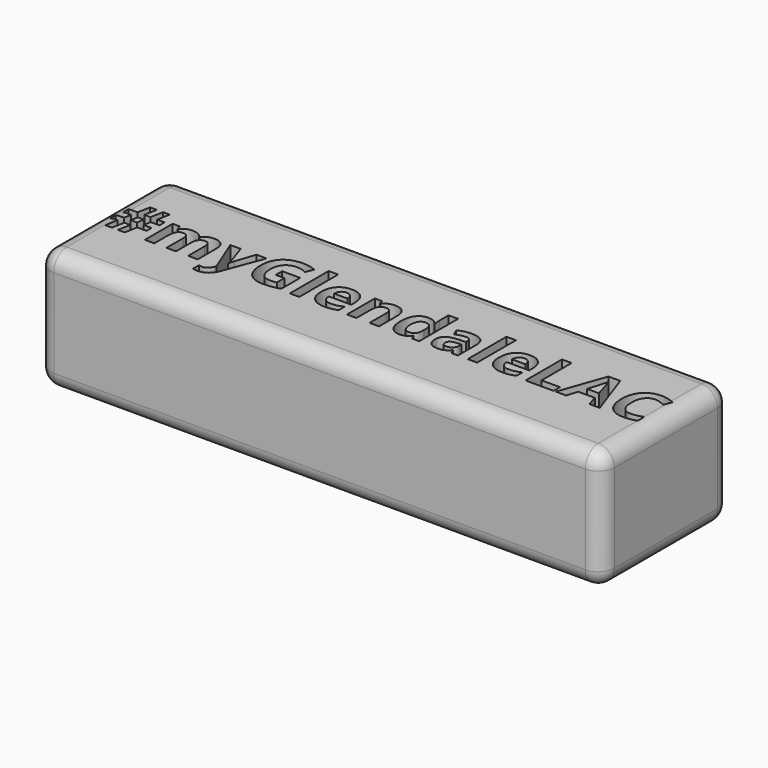
from build123d import *

# Parameters (mm, degrees)
F0_W         = 177.8
F0_H         = 50.8
F1_DEPTH     = 38.1
F2_TEXT_SIZE = 20.1029624608
F3_DEPTH     = 38.1
F4_T1_DEPTH  = 167.64
F4_T3_DEPTH  = 40.64
F4_T5_DEPTH  = 27.94
F4_S9_W      = 5.1816
F4_S9_H      = 5.1816
F4_T10_DEPTH = 5.1816
F4_S15_W     = 5.1816
F4_S15_H     = 5.1816
F4_T16_DEPTH = 5.1816
F4_S21_W     = 5.1816
F4_S21_H     = 5.1816
F4_T22_DEPTH = 5.1816
F4_S27_W     = 5.1816
F4_S27_H     = 5.1816
F4_T28_DEPTH = 5.1816
F4_S33_W     = 5.1816
F4_S33_H     = 5.1816
F4_T34_DEPTH = 5.1816
F4_S39_W     = 5.1816
F4_S39_H     = 5.1816
F4_T40_DEPTH = 5.1816
F4_S45_W     = 5.1816
F4_S45_H     = 5.1816
F4_T46_DEPTH = 5.1816
F4_S51_W     = 5.1816
F4_S51_H     = 5.1816
F4_T52_DEPTH = 5.1816


# Not quite as in the source:
# - a fillet or chamfer that OpenCascade refuses, or shapes differently, is made with other operations: its cross-section is extruded or revolved along the edge and cut away or added
# - Text() gives the source's letters only with a copy of the font that has no kerning and outlines rounded to 1/6400 em; it was checked with that copy


with BuildPart() as f1:
    # F0 (on Top) → F1 (new body)
    with BuildSketch(Plane.XY):
        Rectangle(F0_W, F0_H)
    extrude(amount=F1_DEPTH)

    # F2 (on face) → F3 (cut, through all)
    with BuildSketch(Plane.XY.offset(38.1)):
        with Locations((-85.725, -5.3196763222)):
            Text('#myGlendaleLAC', F2_TEXT_SIZE, font='Open Sans', font_style=FontStyle.BOLD, text_align=(TextAlign.LEFT, TextAlign.BOTTOM))
    extrude(amount=-F3_DEPTH, mode=Mode.SUBTRACT)

    # F4: fillet of radius 5.08 on 12 edges, made by hand

    # F4_s2 → F4_t1 (cut)
    with BuildSketch(Plane.YZ.offset(-83.82)):
        with BuildLine():
            ThreePointArc((25.4, 33.02), (23.9121024484, 36.6121024484), (20.32, 38.1))
            Line((20.32, 38.1), (20.32, 38.2016))
            Line((20.32, 38.2016), (25.5016, 38.2016))
            Line((25.5016, 38.2016), (25.5016, 33.02))
            Line((25.5016, 33.02), (25.4, 33.02))
        make_face()
        with BuildLine():
            ThreePointArc((-25.4, 5.08), (-23.9121024484, 1.4878975516), (-20.32, 0))
            Line((-20.32, 0), (-20.32, -0.1016))
            Line((-20.32, -0.1016), (-25.5016, -0.1016))
            Line((-25.5016, -0.1016), (-25.5016, 5.08))
            Line((-25.5016, 5.08), (-25.4, 5.08))
        make_face()
        with BuildLine():
            ThreePointArc((-25.4, 33.02), (-23.9121024484, 36.6121024484), (-20.32, 38.1))
            Line((-20.32, 38.1), (-20.32, 38.2016))
            Line((-20.32, 38.2016), (-25.5016, 38.2016))
            Line((-25.5016, 38.2016), (-25.5016, 33.02))
            Line((-25.5016, 33.02), (-25.4, 33.02))
        make_face()
        with BuildLine():
            ThreePointArc((25.4, 5.08), (23.9121024484, 1.4878975516), (20.32, 0))
            Line((20.32, 0), (20.32, -0.1016))
            Line((20.32, -0.1016), (25.5016, -0.1016))
            Line((25.5016, -0.1016), (25.5016, 5.08))
            Line((25.5016, 5.08), (25.4, 5.08))
        make_face()
    extrude(amount=F4_T1_DEPTH, mode=Mode.SUBTRACT)

    # F4_s4 → F4_t3 (cut)
    with BuildSketch(Plane.XZ.offset(-20.32)):
        with BuildLine():
            ThreePointArc((-83.82, 38.1), (-87.4121024484, 36.6121024484), (-88.9, 33.02))
            Line((-88.9, 33.02), (-89.0016, 33.02))
            Line((-89.0016, 33.02), (-89.0016, 38.2016))
            Line((-89.0016, 38.2016), (-83.82, 38.2016))
            Line((-83.82, 38.2016), (-83.82, 38.1))
        make_face()
        with BuildLine():
            ThreePointArc((-83.82, 0), (-87.4121024484, 1.4878975516), (-88.9, 5.08))
            Line((-88.9, 5.08), (-89.0016, 5.08))
            Line((-89.0016, 5.08), (-89.0016, -0.1016))
            Line((-89.0016, -0.1016), (-83.82, -0.1016))
            Line((-83.82, -0.1016), (-83.82, 0))
        make_face()
        with BuildLine():
            ThreePointArc((88.9, 5.08), (87.4121024484, 1.4878975516), (83.82, 0))
            Line((83.82, 0), (83.82, -0.1016))
            Line((83.82, -0.1016), (89.0016, -0.1016))
            Line((89.0016, -0.1016), (89.0016, 5.08))
            Line((89.0016, 5.08), (88.9, 5.08))
        make_face()
        with BuildLine():
            ThreePointArc((88.9, 33.02), (87.4121024484, 36.6121024484), (83.82, 38.1))
            Line((83.82, 38.1), (83.82, 38.2016))
            Line((83.82, 38.2016), (89.0016, 38.2016))
            Line((89.0016, 38.2016), (89.0016, 33.02))
            Line((89.0016, 33.02), (88.9, 33.02))
        make_face()
    extrude(amount=F4_T3_DEPTH, mode=Mode.SUBTRACT)

    # F4_s6 → F4_t5 (cut)
    with BuildSketch(Plane.XY.offset(5.08)):
        with BuildLine():
            ThreePointArc((-83.82, 25.4), (-87.4121024484, 23.9121024484), (-88.9, 20.32))
            Line((-88.9, 20.32), (-89.0016, 20.32))
            Line((-89.0016, 20.32), (-89.0016, 25.5016))
            Line((-89.0016, 25.5016), (-83.82, 25.5016))
            Line((-83.82, 25.5016), (-83.82, 25.4))
        make_face()
        with BuildLine():
            ThreePointArc((-83.82, -25.4), (-87.4121024484, -23.9121024484), (-88.9, -20.32))
            Line((-88.9, -20.32), (-89.0016, -20.32))
            Line((-89.0016, -20.32), (-89.0016, -25.5016))
            Line((-89.0016, -25.5016), (-83.82, -25.5016))
            Line((-83.82, -25.5016), (-83.82, -25.4))
        make_face()
        with BuildLine():
            ThreePointArc((88.9, -20.32), (87.4121024484, -23.9121024484), (83.82, -25.4))
            Line((83.82, -25.4), (83.82, -25.5016))
            Line((83.82, -25.5016), (89.0016, -25.5016))
            Line((89.0016, -25.5016), (89.0016, -20.32))
            Line((89.0016, -20.32), (88.9, -20.32))
        make_face()
        with BuildLine():
            ThreePointArc((88.9, 20.32), (87.4121024484, 23.9121024484), (83.82, 25.4))
            Line((83.82, 25.4), (83.82, 25.5016))
            Line((83.82, 25.5016), (89.0016, 25.5016))
            Line((89.0016, 25.5016), (89.0016, 20.32))
            Line((89.0016, 20.32), (88.9, 20.32))
        make_face()
    extrude(amount=F4_T5_DEPTH, mode=Mode.SUBTRACT)


with BuildPart() as f4_tool8:
    # F4_s9 → F4_t10 (new body)
    with BuildSketch(Plane.YZ.offset(83.82)):
        with Locations((22.9108, 35.6108)):
            Rectangle(F4_S9_W, F4_S9_H)
    extrude(amount=F4_T10_DEPTH)

    # F4_s11 → F4_t12 (revolve, cut)
    with BuildSketch(Plane(origin=(83.82, 20.32, 33.02), x_dir=(0, -0.7071067812, -0.7071067812), z_dir=(0, -0.7071067812, 0.7071067812))):
        with BuildLine():
            ThreePointArc((0, -5.08), (5.08, 0), (0, 5.08))
            Line((0, 5.08), (0, -5.08))
        make_face()
    revolve(axis=Axis((83.82, 20.32, 33.02), (1, 0, 0)), mode=Mode.SUBTRACT)


with BuildPart() as f1_1:
    add(f1.part)

    # F4_t7: cut F4_tool8
    add(f4_tool8.part, mode=Mode.SUBTRACT)


with BuildPart() as f4_tool14:
    # F4_s15 → F4_t16 (new body)
    with BuildSketch(Plane.XZ.offset(-20.32)):
        with Locations((-86.4108, 35.6108)):
            Rectangle(F4_S15_W, F4_S15_H)
    extrude(amount=-F4_T16_DEPTH)

    # F4_s17 → F4_t18 (revolve, cut)
    with BuildSketch(Plane(origin=(-83.82, 20.32, 33.02), x_dir=(0.7071067812, 0, -0.7071067812), z_dir=(0.7071067812, 0, 0.7071067812))):
        with BuildLine():
            ThreePointArc((0, -5.08), (5.08, 0), (0, 5.08))
            Line((0, 5.08), (0, -5.08))
        make_face()
    revolve(axis=Axis((-83.82, 20.32, 33.02), (0, 1, 0)), mode=Mode.SUBTRACT)


with BuildPart() as f1_2:
    add(f1_1.part)

    # F4_t13: cut F4_tool14
    add(f4_tool14.part, mode=Mode.SUBTRACT)


with BuildPart() as f4_tool20:
    # F4_s21 → F4_t22 (new body)
    with BuildSketch(Plane.XZ.offset(20.32)):
        with Locations((-86.4108, 35.6108)):
            Rectangle(F4_S21_W, F4_S21_H)
    extrude(amount=F4_T22_DEPTH)

    # F4_s23 → F4_t24 (revolve, cut)
    with BuildSketch(Plane(origin=(-83.82, -20.32, 33.02), x_dir=(0.7071067812, 0, -0.7071067812), z_dir=(-0.7071067812, 0, -0.7071067812))):
        with BuildLine():
            ThreePointArc((0, -5.08), (5.08, 0), (0, 5.08))
            Line((0, 5.08), (0, -5.08))
        make_face()
    revolve(axis=Axis((-83.82, -20.32, 33.02), (0, -1, 0)), mode=Mode.SUBTRACT)


with BuildPart() as f1_3:
    add(f1_2.part)

    # F4_t19: cut F4_tool20
    add(f4_tool20.part, mode=Mode.SUBTRACT)


with BuildPart() as f4_tool26:
    # F4_s27 → F4_t28 (new body)
    with BuildSketch(Plane.XZ.offset(-20.32)):
        with Locations((-86.4108, 2.4892)):
            Rectangle(F4_S27_W, F4_S27_H)
    extrude(amount=-F4_T28_DEPTH)

    # F4_s29 → F4_t30 (revolve, cut)
    with BuildSketch(Plane(origin=(-83.82, 20.32, 5.08), x_dir=(0.7071067812, 0, 0.7071067812), z_dir=(-0.7071067812, 0, 0.7071067812))):
        with BuildLine():
            ThreePointArc((0, -5.08), (5.08, 0), (0, 5.08))
            Line((0, 5.08), (0, -5.08))
        make_face()
    revolve(axis=Axis((-83.82, 20.32, 5.08), (0, 1, 0)), mode=Mode.SUBTRACT)


with BuildPart() as f1_4:
    add(f1_3.part)

    # F4_t25: cut F4_tool26
    add(f4_tool26.part, mode=Mode.SUBTRACT)


with BuildPart() as f4_tool32:
    # F4_s33 → F4_t34 (new body)
    with BuildSketch(Plane.XZ.offset(20.32)):
        with Locations((-86.4108, 2.4892)):
            Rectangle(F4_S33_W, F4_S33_H)
    extrude(amount=F4_T34_DEPTH)

    # F4_s35 → F4_t36 (revolve, cut)
    with BuildSketch(Plane(origin=(-83.82, -20.32, 5.08), x_dir=(0.7071067812, 0, 0.7071067812), z_dir=(0.7071067812, 0, -0.7071067812))):
        with BuildLine():
            ThreePointArc((0, -5.08), (5.08, 0), (0, 5.08))
            Line((0, 5.08), (0, -5.08))
        make_face()
    revolve(axis=Axis((-83.82, -20.32, 5.08), (0, -1, 0)), mode=Mode.SUBTRACT)


with BuildPart() as f1_5:
    add(f1_4.part)

    # F4_t31: cut F4_tool32
    add(f4_tool32.part, mode=Mode.SUBTRACT)


with BuildPart() as f4_tool38:
    # F4_s39 → F4_t40 (new body)
    with BuildSketch(Plane.YZ.offset(83.82)):
        with Locations((-22.9108, 2.4892)):
            Rectangle(F4_S39_W, F4_S39_H)
    extrude(amount=F4_T40_DEPTH)

    # F4_s41 → F4_t42 (revolve, cut)
    with BuildSketch(Plane(origin=(83.82, -20.32, 5.08), x_dir=(0, 0.7071067812, 0.7071067812), z_dir=(0, 0.7071067812, -0.7071067812))):
        with BuildLine():
            ThreePointArc((0, -5.08), (5.08, 0), (0, 5.08))
            Line((0, 5.08), (0, -5.08))
        make_face()
    revolve(axis=Axis((83.82, -20.32, 5.08), (1, 0, 0)), mode=Mode.SUBTRACT)


with BuildPart() as f1_6:
    add(f1_5.part)

    # F4_t37: cut F4_tool38
    add(f4_tool38.part, mode=Mode.SUBTRACT)


with BuildPart() as f4_tool44:
    # F4_s45 → F4_t46 (new body)
    with BuildSketch(Plane.YZ.offset(83.82)):
        with Locations((-22.9108, 35.6108)):
            Rectangle(F4_S45_W, F4_S45_H)
    extrude(amount=F4_T46_DEPTH)

    # F4_s47 → F4_t48 (revolve, cut)
    with BuildSketch(Plane(origin=(83.82, -20.32, 33.02), x_dir=(0, 0.7071067812, -0.7071067812), z_dir=(0, -0.7071067812, -0.7071067812))):
        with BuildLine():
            ThreePointArc((0, -5.08), (5.08, 0), (0, 5.08))
            Line((0, 5.08), (0, -5.08))
        make_face()
    revolve(axis=Axis((83.82, -20.32, 33.02), (1, 0, 0)), mode=Mode.SUBTRACT)


with BuildPart() as f1_7:
    add(f1_6.part)

    # F4_t43: cut F4_tool44
    add(f4_tool44.part, mode=Mode.SUBTRACT)


with BuildPart() as f4_tool50:
    # F4_s51 → F4_t52 (new body)
    with BuildSketch(Plane.YZ.offset(83.82)):
        with Locations((22.9108, 2.4892)):
            Rectangle(F4_S51_W, F4_S51_H)
    extrude(amount=F4_T52_DEPTH)

    # F4_s53 → F4_t54 (revolve, cut)
    with BuildSketch(Plane(origin=(83.82, 20.32, 5.08), x_dir=(0, -0.7071067812, 0.7071067812), z_dir=(0, 0.7071067812, 0.7071067812))):
        with BuildLine():
            ThreePointArc((0, -5.08), (5.08, 0), (0, 5.08))
            Line((0, 5.08), (0, -5.08))
        make_face()
    revolve(axis=Axis((83.82, 20.32, 5.08), (1, 0, 0)), mode=Mode.SUBTRACT)


with BuildPart() as f1_8:
    add(f1_7.part)

    # F4_t49: cut F4_tool50
    add(f4_tool50.part, mode=Mode.SUBTRACT)


solid = f1_8.part
